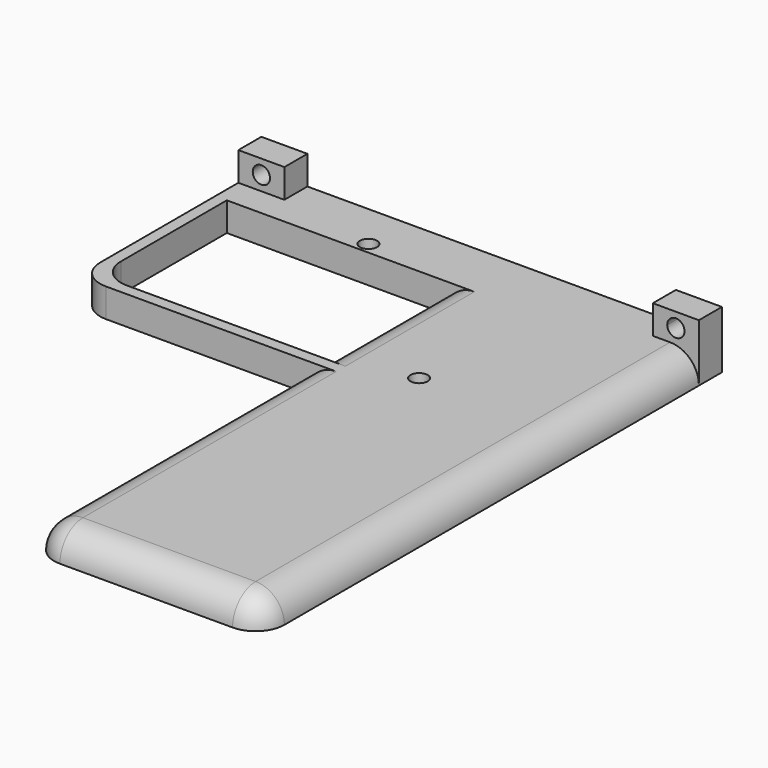
from build123d import *

# Parameters (mm, degrees)
F0_W     = 38
F0_H     = 10
F1_DEPTH = 5
F2_R     = 1.5
F3_DEPTH = 5
F4_W     = 8
F4_H     = 5
F5_DEPTH = 5
F6_R     = 1.5
F7_DEPTH = 5
F8_R     = 4.99999


# Not quite as in the source:
# - a fillet or chamfer is up to 0.001 mm smaller than in the source, because OpenCascade refuses the exact size
# - a feature names something its author has since deleted; it is built from what else it names


with BuildPart() as f1:
    # F0 (on Top) → F1 (new body)
    with BuildSketch(Plane.XY):
        Polygon((20, -50), (20, 50), (-20, 50), (-20, 40), (-20, 12), (-20, 10), (-20, -50), align=None)
        with Locations((-39, 45)):
            Rectangle(F0_W, F0_H)
        Polygon((-58, 40), (-58, 50), (-60, 50), (-60, 10), (-20, 10), (-20, 12), (-58, 12), align=None)
    extrude(amount=F1_DEPTH)

    # F2 (on face) → F3 (cut)
    with BuildSketch(Plane.XY.offset(5)):
        with Locations((-35, 42)):
            Circle(F2_R)
        with Locations((-5, 15.5)):
            Circle(F2_R)
    extrude(amount=-F3_DEPTH, mode=Mode.SUBTRACT)

    # F4 (on face) → F5 (join)
    with BuildSketch(Plane.XY.offset(5)):
        with Locations((16, 47.5)):
            Rectangle(F4_W, F4_H)
        with Locations((-56, 47.5)):
            Rectangle(F4_W, F4_H)
    extrude(amount=F5_DEPTH)

    # F6 (on face) → F7 (cut)
    with BuildSketch(Plane(origin=(0, 50, 0), x_dir=(-1, 0, 0), z_dir=(0, 1, 0))):
        with BuildLine():
            ThreePointArc((-14.5, 7.5), (-14.9393398282, 8.5606601718), (-16, 9))
            ThreePointArc((-16, 9), (-17.0606601718, 6.4393398282), (-14.5, 7.5))
        make_face()
        with Locations((56, 7.5)):
            Circle(F6_R)
    extrude(amount=-F7_DEPTH, mode=Mode.SUBTRACT)

    # F8 (radius 5 in the source; OpenCascade refuses exactly that, so slightly less here)
    f8_edges = [f1.edges().sort_by_distance(p)[0] for p in [
        (-60, 10, 2.5),
        (-58, 12, 2.5),
        (-20, -20, 5),
        (-20, 26, 5),
        (0, -50, 5),
        (20, -2.5, 5),
        (-20, -50, 2.5),
        (20, -50, 2.5),
    ]]
    fillet(f8_edges, radius=F8_R)


solid = f1.part
